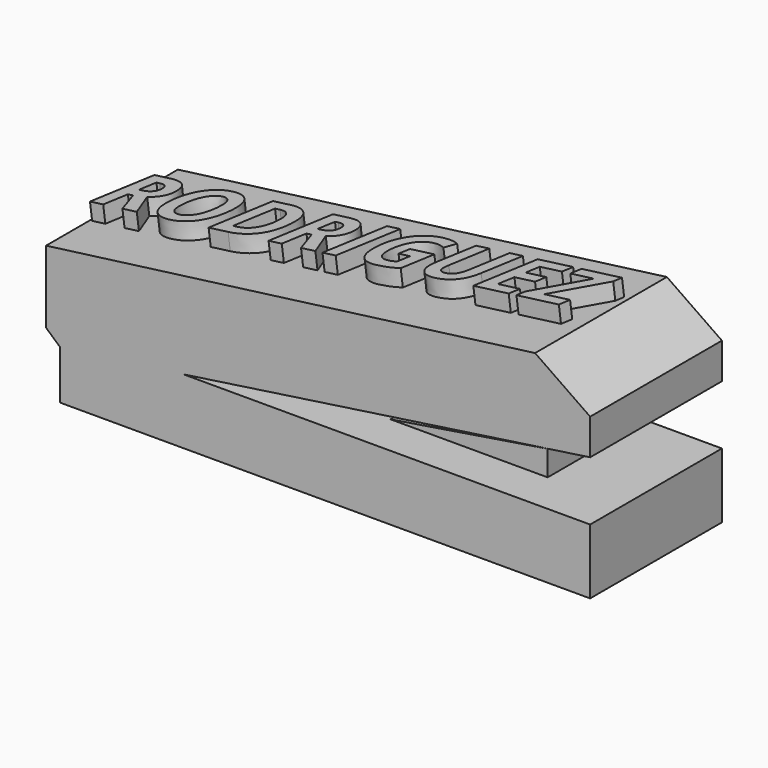
from build123d import *

# Parameters (mm, degrees)
F2_DEPTH     = 25.4
F3_DEPTH     = 25.4
F4_TEXT_SIZE = 13.7782236799
F5_DEPTH     = 2.54


# Not quite as in the source:
# - Text() gives the source's letters only with a copy of the font that has no kerning and outlines rounded to 1/6400 em; it was checked with that copy


with BuildPart() as f2:
    # F0 (on Front) → F2 (new body)
    with BuildSketch(Plane.XZ):
        Polygon((-50.915453583, 4.1217273101), (-50.915453583, 0), (30.7917296886, 0), (30.7917296886, 4.1217273101), (30.7917296886, 10.0313192), (-31.9260764721, 10.0313192), (30.7917296886, 19.1539097577), (30.7917296886, 24.6744078071), (22.3058201373, 30.5492728949), (-53.0975461006, 20.6086356193), (-53.0975461006, 9.4557274133), (-50.915453583, 7.5160907581), align=None)
    extrude(amount=F2_DEPTH)

    # F4 (on face) → F5 (join)
    with BuildSketch(Plane(origin=(-3.5775463136, 0, 27.1369960935), x_dir=(0.9914217125, 0, 0.1307019053), z_dir=(-0.1307019053, 0, 0.9914217125))):
        with Locations((-49.9484721427, -16.9650464065)):
            Text('RODRIGUEZ', F4_TEXT_SIZE, font='Open Sans', font_style=FontStyle.BOLDITALIC, text_align=(TextAlign.LEFT, TextAlign.BOTTOM))
    extrude(amount=F5_DEPTH)


with BuildPart() as f3:
    # F1 (on Front) → F3 (new body)
    with BuildSketch(Plane.XZ):
        Polygon((24.2454558611, 14.3048176542), (24.2454558611, 18.1840918958), (0, 14.3048176542), align=None)
    extrude(amount=F3_DEPTH)


solid = Compound([f2.part, f3.part])
